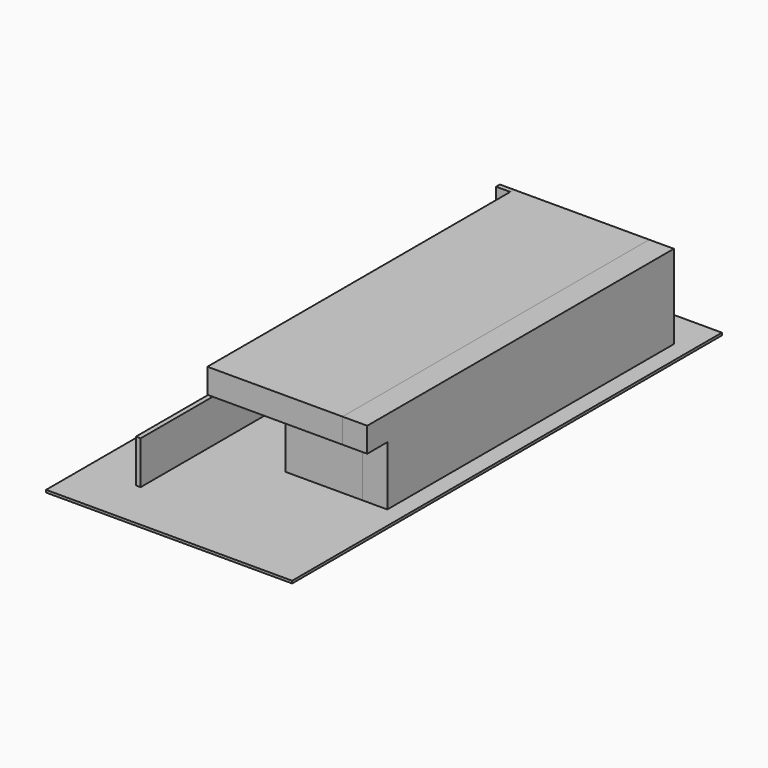
from build123d import *

# Parameters (mm, degrees)
F0_W      = 3962.4
F0_H      = 100.584
F0_W_2    = 3657.6
F1_DEPTH  = 3048
F0_H_2    = 6705.6
F2_W      = 7680.96
F2_H      = 243.84
F3_DEPTH  = 2212.848
F2_W_2    = 243.84
F2_H_2    = 22860
F4_W      = 6952.488
F4_H      = 19720.56
F5_DEPTH  = 1270
F7_DEPTH  = 1270
F8_W      = 12660.7222557068
F8_H      = 27640.1681900024
F9_DEPTH  = 127
F10_W     = 7680.96
F10_H     = 243.84
F11_DEPTH = 2105.152
F12_W     = 203.2
F12_H     = 1042.4841030922
F13_DEPTH = 1695.45
F12_H_2   = 263.5509208527
F12_H_3   = 1295.4
F12_W_2   = 76.2
F12_H_4   = 1074.7200767822
F12_W_3   = 92.6412559891
F12_H_5   = 288.721465332
F12_H_6   = 1012.3699176077
F12_H_7   = 378.1757420269
F12_H_8   = 1066.9633667297
F12_H_9   = 254.1736595459
F12_W_4   = 749.3
F12_H_10  = 1600.2
F16_W     = 673.1
F16_H     = 50.8
F16_W_2   = 647.7
F17_DEPTH = 10558.3631044312
F18_W     = 749.3
F18_H     = 1600.2
F19_DEPTH = 50.8


with BuildPart() as f1:
    # F0 (on Top) → F1 (new body)
    with BuildSketch(Plane.XY):
        with Locations((1981.2, 50.292)):
            Rectangle(F0_W, F0_H)
        with Locations((-1828.8, 50.292)):
            Rectangle(F0_W_2, F0_H)
    extrude(amount=F1_DEPTH)


with BuildPart() as f1b:
    # F0 (on Top) → F1, piece 2 (new body)
    with BuildSketch(Plane.XY):
        with Locations((1981.2, -5791.2)):
            Rectangle(F0_W, F0_H_2)
    extrude(amount=F1_DEPTH)


with BuildPart() as f3:
    # F2 (on Top) → F3 (new body)
    with BuildSketch(Plane.XY):
        with Locations((121.92, 9162.288)):
            Rectangle(F2_W, F2_H)
    extrude(amount=F3_DEPTH)

    # F10 (on face) → F11 (join, through all)
    with BuildSketch(Plane.XY.offset(2212.848)):
        with Locations((121.92, 9162.288)):
            Rectangle(F10_W, F10_H)
    extrude(amount=F11_DEPTH)


with BuildPart() as f3b:
    # F2 (on Top) → F3, piece 2 (new body)
    with BuildSketch(Plane.XY):
        with Locations((-3840.48, -2389.632)):
            Rectangle(F2_W_2, F2_H_2)
    extrude(amount=F3_DEPTH)


with BuildPart() as f5:
    # F4 (on face) → F5 (new body)
    with BuildSketch(Plane.XY.offset(3048)):
        with Locations((486.156, -576.072)):
            Rectangle(F4_W, F4_H)
    extrude(amount=F5_DEPTH)


with BuildPart() as f7:
    # F6 (on face) → F7 (new body)
    with BuildSketch(Plane.YZ.offset(3962.4)):
        Polygon((-9144, 3048), (-9144, 0), (9284.208, 0), (9284.208, 4318), (-9144, 4318), (-10436.352, 4318), (-10436.352, 3048), align=None)
    extrude(amount=F7_DEPTH)


with BuildPart() as f9:
    # F8 (on Top) → F9 (new body)
    with BuildSketch(Plane.XY):
        with Locations((-212.5051021576, -2551.5379905701)):
            Rectangle(F8_W, F8_H)
    extrude(amount=-F9_DEPTH)


with BuildPart() as f13:
    # F12 (on Top) → F13 (new body)
    with BuildSketch(Plane.XY):
        Polygon((-2499.36, 2005.584), (-2499.36, 710.184), (-1724.66, 710.184), (-1724.66, 2005.584), (-1800.86, 2005.584), (-1800.86, 963.0998969078), (-2004.06, 963.0998969078), (-2004.06, 2005.584), align=None)
        with Locations((-1902.46, 1484.3419484539)):
            Rectangle(F12_W, F12_H)
    extrude(amount=F13_DEPTH)


with BuildPart() as f13b:
    # F12 (on Top) → F13, piece 2 (new body)
    with BuildSketch(Plane.XY):
        Polygon((-2499.36, 2107.184), (-2004.06, 2107.184), (-2004.06, 3402.584), (-2219.96, 3402.584), (-2219.96, 3139.0330791473), (-2423.16, 3139.0330791473), (-2423.16, 3402.584), (-2499.36, 3402.584), align=None)
        with Locations((-2321.56, 3270.8085395737)):
            Rectangle(F12_W, F12_H_2)
        with Locations((-1902.46, 2754.884)):
            Rectangle(F12_W, F12_H_3)
        with Locations((-1762.76, 2754.884)):
            Rectangle(F12_W_2, F12_H_3)
    extrude(amount=F13_DEPTH)


with BuildPart() as f13c:
    # F12 (on Top) → F13, piece 3 (new body)
    with BuildSketch(Plane.XY):
        Polygon((-2499.36, 6830.568), (-2499.36, 5535.168), (-2423.16, 5535.168), (-2423.16, 6609.8880767822), (-2219.96, 6609.8880767822), (-2219.96, 5535.168), (-2020.5012559891, 5535.168), (-2020.5012559891, 6830.568), align=None)
        with Locations((-2321.56, 6072.5280383911)):
            Rectangle(F12_W, F12_H_4)
        with Locations((-1770.9806279945, 6182.868)):
            Rectangle(F12_W_3, F12_H_3)
        with Locations((-1918.9012559891, 6182.868)):
            Rectangle(F12_W, F12_H_3)
    extrude(amount=F13_DEPTH)


with BuildPart() as f13d:
    # F12 (on Top) → F13, piece 4 (new body)
    with BuildSketch(Plane.XY):
        Polygon((-2499.36, 7440.168), (-2020.5012559891, 7440.168), (-2020.5012559891, 7728.889465332), (-1817.3012559891, 7728.889465332), (-1817.3012559891, 7440.168), (-1724.66, 7440.168), (-1724.66, 8735.568), (-2499.36, 8735.568), align=None)
        with Locations((-1918.9012559891, 7584.528732666)):
            Rectangle(F12_W, F12_H_5)
    extrude(amount=F13_DEPTH)


with BuildPart() as f13e:
    # F12 (on Top) → F13, piece 5 (new body)
    with BuildSketch(Plane.XY):
        Polygon((459.74, 993.2140823923), (459.74, 2005.584), (-35.56, 2005.584), (-35.56, 710.184), (739.14, 710.184), (739.14, 2005.584), (662.94, 2005.584), (662.94, 993.2140823923), align=None)
        with Locations((561.34, 1499.3990411962)):
            Rectangle(F12_W, F12_H_6)
    extrude(amount=F13_DEPTH)


with BuildPart() as f13f:
    # F12 (on Top) → F13, piece 6 (new body)
    with BuildSketch(Plane.XY):
        Polygon((40.64, 3402.584), (-35.56, 3402.584), (-35.56, 2107.184), (459.74, 2107.184), (459.74, 3402.584), (243.84, 3402.584), (243.84, 3024.4082579731), (40.64, 3024.4082579731), align=None)
        with Locations((142.24, 3213.4961289866)):
            Rectangle(F12_W, F12_H_7)
        with Locations((701.04, 2754.884)):
            Rectangle(F12_W_2, F12_H_3)
        with Locations((561.34, 2754.884)):
            Rectangle(F12_W, F12_H_3)
    extrude(amount=F13_DEPTH)


with BuildPart() as f13g:
    # F12 (on Top) → F13, piece 7 (new body)
    with BuildSketch(Plane.XY):
        with Locations((142.24, 6068.6496833649)):
            Rectangle(F12_W, F12_H_8)
        Polygon((459.74, 6830.568), (-35.56, 6830.568), (-35.56, 5535.168), (40.64, 5535.168), (40.64, 6602.1313667297), (243.84, 6602.1313667297), (243.84, 5535.168), (459.74, 5535.168), align=None)
        with Locations((561.34, 6182.868)):
            Rectangle(F12_W, F12_H_3)
        with Locations((701.04, 6182.868)):
            Rectangle(F12_W_2, F12_H_3)
    extrude(amount=F13_DEPTH)


with BuildPart() as f13h:
    # F12 (on Top) → F13, piece 8 (new body)
    with BuildSketch(Plane.XY):
        Polygon((-35.56, 7440.168), (459.74, 7440.168), (459.74, 7694.3416595459), (662.94, 7694.3416595459), (662.94, 7440.168), (739.14, 7440.168), (739.14, 8735.568), (-35.56, 8735.568), align=None)
        with Locations((561.34, 7567.2548297729)):
            Rectangle(F12_W, F12_H_9)
    extrude(amount=F13_DEPTH)


with BuildPart() as f13i:
    # F12 (on Top) → F13, piece 9 (new body)
    with BuildSketch(Plane.XY):
        with Locations((3040.2774199486, 7831.310899353)):
            Rectangle(F12_W_4, F12_H_10)
    extrude(amount=F13_DEPTH)


with BuildPart() as f17_tool:
    # F16 (on face) → F17 (new body, through all)
    with BuildSketch(Plane.XZ.offset(-710.184)):
        with Locations((351.79, 25.4)):
            Rectangle(F16_W, F16_H)
        with Locations((-2112.01, 25.4)):
            Rectangle(F16_W_2, F16_H)
    extrude(amount=-F17_DEPTH)


with BuildPart() as f13_1:
    add(f13.part)

    # F17: cut by f17_tool
    add(f17_tool.part, mode=Mode.SUBTRACT)


with BuildPart() as f13b_1:
    add(f13b.part)

    # F17: cut by f17_tool
    add(f17_tool.part, mode=Mode.SUBTRACT)


with BuildPart() as f13c_1:
    add(f13c.part)

    # F17: cut by f17_tool
    add(f17_tool.part, mode=Mode.SUBTRACT)


with BuildPart() as f13d_1:
    add(f13d.part)

    # F17: cut by f17_tool
    add(f17_tool.part, mode=Mode.SUBTRACT)


with BuildPart() as f13e_1:
    add(f13e.part)

    # F17: cut by f17_tool
    add(f17_tool.part, mode=Mode.SUBTRACT)


with BuildPart() as f13f_1:
    add(f13f.part)

    # F17: cut by f17_tool
    add(f17_tool.part, mode=Mode.SUBTRACT)


with BuildPart() as f13g_1:
    add(f13g.part)

    # F17: cut by f17_tool
    add(f17_tool.part, mode=Mode.SUBTRACT)


with BuildPart() as f13h_1:
    add(f13h.part)

    # F17: cut by f17_tool
    add(f17_tool.part, mode=Mode.SUBTRACT)


with BuildPart() as f19:
    # F18 (on face) → F19 (new body)
    with BuildSketch(Plane.XY):
        with Locations((3040.2774199486, 7831.310899353)):
            Rectangle(F18_W, F18_H)
    extrude(amount=F19_DEPTH)


with BuildPart() as f19b:
    # F18 (on face) → F19, piece 2 (new body)
    with BuildSketch(Plane.XY):
        with BuildLine():
            Line((-2004.06, 3910.584), (-2004.06, 963.0998969078))
            Line((-2004.06, 963.0998969078), (-1800.86, 963.0998969078))
            Line((-1800.86, 963.0998969078), (-1800.86, 3910.584))
            ThreePointArc((-1800.86, 3910.584), (-1795.0596203774, 3939.7444775462), (-1778.5415367264, 3964.4655367264))
            Line((-1778.5415367264, 3964.4655367264), (-1922.2256346635, 4108.1496346635))
            ThreePointArc((-1922.2256346635, 4108.1496346635), (-1982.7919413837, 4017.5057510028), (-2004.06, 3910.584))
        make_face()
        with BuildLine():
            ThreePointArc((-1724.66, 4189.984), (-1831.5817510028, 4168.7159413837), (-1922.2256346635, 4108.1496346635))
            Line((-1922.2256346635, 4108.1496346635), (-1778.5415367264, 3964.4655367264))
            ThreePointArc((-1778.5415367264, 3964.4655367264), (-1753.8204775462, 3980.9836203774), (-1724.66, 3986.784))
            Line((-1724.66, 3986.784), (3872.3020553589, 3986.784))
            Line((3872.3020553589, 3986.784), (3872.3020553589, 4189.984))
            Line((3872.3020553589, 4189.984), (-1724.66, 4189.984))
        make_face()
    extrude(amount=F19_DEPTH)


with BuildPart() as f19c:
    # F18 (on face) → F19, piece 3 (new body)
    with BuildSketch(Plane.XY):
        with BuildLine():
            Line((-2423.16, 4139.184), (-2423.16, 3139.0330791473))
            Line((-2423.16, 3139.0330791473), (-2219.96, 3139.0330791473))
            Line((-2219.96, 3139.0330791473), (-2219.96, 4139.184))
            ThreePointArc((-2219.96, 4139.184), (-2214.1596203774, 4168.3444775462), (-2197.6415367264, 4193.0655367264))
            Line((-2197.6415367264, 4193.0655367264), (-2341.3256346635, 4336.7496346635))
            ThreePointArc((-2341.3256346635, 4336.7496346635), (-2401.8919413836, 4246.1057510028), (-2423.16, 4139.184))
        make_face()
        with BuildLine():
            ThreePointArc((-2143.76, 4418.584), (-2250.6817510028, 4397.3159413836), (-2341.3256346635, 4336.7496346635))
            Line((-2341.3256346635, 4336.7496346635), (-2197.6415367264, 4193.0655367264))
            ThreePointArc((-2197.6415367264, 4193.0655367264), (-2172.9204775462, 4209.5836203774), (-2143.76, 4215.384))
            Line((-2143.76, 4215.384), (3879.269361496, 4215.384))
            Line((3879.269361496, 4215.384), (3879.269361496, 4418.584))
            Line((3879.269361496, 4418.584), (-2143.76, 4418.584))
        make_face()
    extrude(amount=F19_DEPTH)


with BuildPart() as f19d:
    # F18 (on face) → F19, piece 4 (new body)
    with BuildSketch(Plane.XY):
        with BuildLine():
            Line((459.74, 3453.384), (459.74, 993.2140823923))
            Line((459.74, 993.2140823923), (662.94, 993.2140823923))
            Line((662.94, 993.2140823923), (662.94, 3453.384))
            ThreePointArc((662.94, 3453.384), (668.7403796226, 3482.5444775462), (685.2584632736, 3507.2655367264))
            Line((685.2584632736, 3507.2655367264), (541.5743653365, 3650.9496346635))
            ThreePointArc((541.5743653365, 3650.9496346635), (481.0080586163, 3560.3057510028), (459.74, 3453.384))
        make_face()
        with BuildLine():
            ThreePointArc((739.14, 3732.784), (632.2182489972, 3711.5159413837), (541.5743653365, 3650.9496346635))
            Line((541.5743653365, 3650.9496346635), (685.2584632736, 3507.2655367264))
            ThreePointArc((685.2584632736, 3507.2655367264), (709.9795224538, 3523.7836203774), (739.14, 3529.584))
            Line((739.14, 3529.584), (3914.3819808962, 3529.584))
            Line((3914.3819808962, 3529.584), (3914.3819808962, 3732.784))
            Line((3914.3819808962, 3732.784), (739.14, 3732.784))
        make_face()
    extrude(amount=F19_DEPTH)


with BuildPart() as f19e:
    # F18 (on face) → F19, piece 5 (new body)
    with BuildSketch(Plane.XY):
        with BuildLine():
            Line((40.64, 3681.984), (40.64, 3024.4082579731))
            Line((40.64, 3024.4082579731), (243.84, 3024.4082579731))
            Line((243.84, 3024.4082579731), (243.84, 3681.984))
            ThreePointArc((243.84, 3681.984), (249.6403796226, 3711.1444775462), (266.1584632736, 3735.8655367264))
            Line((266.1584632736, 3735.8655367264), (122.4743653365, 3879.5496346635))
            ThreePointArc((122.4743653365, 3879.5496346635), (61.9080586164, 3788.9057510028), (40.64, 3681.984))
        make_face()
        with BuildLine():
            ThreePointArc((320.04, 3961.384), (213.1182489972, 3940.1159413836), (122.4743653365, 3879.5496346635))
            Line((122.4743653365, 3879.5496346635), (266.1584632736, 3735.8655367264))
            ThreePointArc((266.1584632736, 3735.8655367264), (290.8795224538, 3752.3836203774), (320.04, 3758.184))
            Line((320.04, 3758.184), (3899.5864391327, 3758.184))
            Line((3899.5864391327, 3758.184), (3899.5864391327, 3961.384))
            Line((3899.5864391327, 3961.384), (320.04, 3961.384))
        make_face()
    extrude(amount=F19_DEPTH)


with BuildPart() as f19f:
    # F18 (on face) → F19, piece 6 (new body)
    with BuildSketch(Plane.XY):
        with BuildLine():
            ThreePointArc((-2197.6415367264, 4694.9024632736), (-2214.1596203774, 4719.6235224538), (-2219.96, 4748.784))
            Line((-2219.96, 4748.784), (-2219.96, 6609.8880767822))
            Line((-2219.96, 6609.8880767822), (-2423.16, 6609.8880767822))
            Line((-2423.16, 6609.8880767822), (-2423.16, 4748.784))
            ThreePointArc((-2423.16, 4748.784), (-2401.8919413836, 4641.8622489972), (-2341.3256346635, 4551.2183653365))
            Line((-2341.3256346635, 4551.2183653365), (-2197.6415367264, 4694.9024632736))
        make_face()
        with BuildLine():
            ThreePointArc((-2143.76, 4672.584), (-2172.9204775462, 4678.3843796226), (-2197.6415367264, 4694.9024632736))
            Line((-2197.6415367264, 4694.9024632736), (-2341.3256346635, 4551.2183653365))
            ThreePointArc((-2341.3256346635, 4551.2183653365), (-2250.6817510028, 4490.6520586164), (-2143.76, 4469.384))
            Line((-2143.76, 4469.384), (3879.269361496, 4469.384))
            Line((3879.269361496, 4469.384), (3879.269361496, 4672.584))
            Line((3879.269361496, 4672.584), (87.7069517879, 4672.584))
            Line((87.7069517879, 4672.584), (-547.3446624273, 4865.5679513469))
            Line((-547.3446624273, 4865.5679513469), (-1383.2707508076, 5119.5950508118))
            Line((-1383.2707508076, 5119.5950508118), (-1575.0844478607, 5119.5950508118))
            ThreePointArc((-1575.0844478607, 5119.5950508118), (-1667.7768073718, 5138.0327074801), (-1746.3575954056, 5190.5387113952))
            Line((-1746.3575954056, 5190.5387113952), (-1890.0416933427, 5046.8546134581))
            ThreePointArc((-1890.0416933427, 5046.8546134581), (-1814.5188916731, 4986.2226151118), (-1727.6759147644, 4943.3480287332))
            ThreePointArc((-1727.6759147644, 4943.3480287332), (-1652.5612488896, 4923.1850491512), (-1575.0844478607, 4916.3950508118))
            Line((-1575.0844478607, 4916.3950508118), (-1413.4639972965, 4916.3950508118))
            Line((-1413.4639972965, 4916.3950508118), (-611.1558245137, 4672.584))
            Line((-611.1558245137, 4672.584), (-2143.76, 4672.584))
        make_face()
        with BuildLine():
            ThreePointArc((-2020.5012559891, 5361.8118589401), (-1986.595920327, 5191.3582259725), (-1890.0416933427, 5046.8546134581))
            Line((-1890.0416933427, 5046.8546134581), (-1746.3575954056, 5190.5387113952))
            ThreePointArc((-1746.3575954056, 5190.5387113952), (-1798.8635993207, 5269.119499429), (-1817.3012559891, 5361.8118589401))
            Line((-1817.3012559891, 5361.8118589401), (-1817.3012559891, 7728.889465332))
            Line((-1817.3012559891, 7728.889465332), (-2020.5012559891, 7728.889465332))
            Line((-2020.5012559891, 7728.889465332), (-2020.5012559891, 5361.8118589401))
        make_face()
    extrude(amount=F19_DEPTH)


with BuildPart() as f19g:
    # F18 (on face) → F19, piece 7 (new body)
    with BuildSketch(Plane.XY):
        with BuildLine():
            ThreePointArc((685.2584632736, 5380.7024632736), (668.7403796226, 5405.4235224538), (662.94, 5434.584))
            Line((662.94, 5434.584), (662.94, 7694.3416595459))
            Line((662.94, 7694.3416595459), (459.74, 7694.3416595459))
            Line((459.74, 7694.3416595459), (459.74, 5434.584))
            ThreePointArc((459.74, 5434.584), (481.0080586163, 5327.6622489972), (541.5743653365, 5237.0183653365))
            Line((541.5743653365, 5237.0183653365), (685.2584632736, 5380.7024632736))
        make_face()
        with BuildLine():
            ThreePointArc((739.14, 5358.384), (709.9795224538, 5364.1843796226), (685.2584632736, 5380.7024632736))
            Line((685.2584632736, 5380.7024632736), (541.5743653365, 5237.0183653365))
            ThreePointArc((541.5743653365, 5237.0183653365), (632.2182489972, 5176.4520586163), (739.14, 5155.184))
            Line((739.14, 5155.184), (3914.3819808962, 5155.184))
            Line((3914.3819808962, 5155.184), (3914.3819808962, 5358.384))
            Line((3914.3819808962, 5358.384), (739.14, 5358.384))
        make_face()
    extrude(amount=F19_DEPTH)


with BuildPart() as f19h:
    # F18 (on face) → F19, piece 8 (new body)
    with BuildSketch(Plane.XY):
        with BuildLine():
            ThreePointArc((266.1584632736, 5152.1024632736), (249.6403796226, 5176.8235224538), (243.84, 5205.984))
            Line((243.84, 5205.984), (243.84, 6602.1313667297))
            Line((243.84, 6602.1313667297), (40.64, 6602.1313667297))
            Line((40.64, 6602.1313667297), (40.64, 5205.984))
            ThreePointArc((40.64, 5205.984), (61.9080586164, 5099.0622489972), (122.4743653365, 5008.4183653365))
            Line((122.4743653365, 5008.4183653365), (266.1584632736, 5152.1024632736))
        make_face()
        with BuildLine():
            ThreePointArc((320.04, 5129.784), (290.8795224538, 5135.5843796226), (266.1584632736, 5152.1024632736))
            Line((266.1584632736, 5152.1024632736), (122.4743653365, 5008.4183653365))
            ThreePointArc((122.4743653365, 5008.4183653365), (213.1182489972, 4947.8520586164), (320.04, 4926.584))
            Line((320.04, 4926.584), (3899.5864391327, 4926.584))
            Line((3899.5864391327, 4926.584), (3899.5864391327, 5129.784))
            Line((3899.5864391327, 5129.784), (320.04, 5129.784))
        make_face()
    extrude(amount=F19_DEPTH)


solid = Compound([f1.part, f1b.part, f3.part, f3b.part, f5.part, f7.part, f9.part, f13i.part, f13_1.part, f13b_1.part, f13c_1.part, f13d_1.part, f13e_1.part, f13f_1.part, f13g_1.part, f13h_1.part, f19.part, f19b.part, f19c.part, f19d.part, f19e.part, f19f.part, f19g.part, f19h.part])
